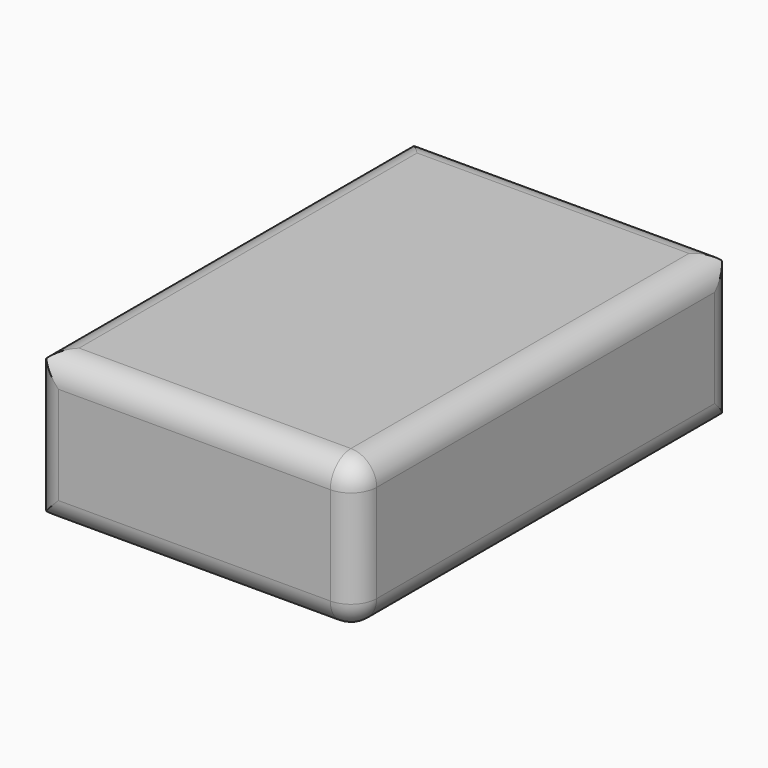
from build123d import *

# Parameters (mm, degrees)
F0_W        = 63.7673679739
F0_H        = 29.4773685746
F1_DEPTH    = 93.472
F2_R        = 5.08
F3_T1_DEPTH = 113.792
F3_T3_DEPTH = 54.8773685746
F4_T1_DEPTH = 79.007367974


# Not quite as in the source:
# - a fillet or chamfer that OpenCascade refuses, or shapes differently, is made with other operations: its cross-section is extruded or revolved along the edge and cut away or added
# - the program builds the solid bodies; features that only make, move or delete a surface that nothing else refers to are left out


with BuildPart() as f1:
    # F0 (on Front) → F1 (new body)
    with BuildSketch(Plane.XZ):
        with Locations((-3.0078953132, 7.5197371189)):
            Rectangle(F0_W, F0_H)
    extrude(amount=F1_DEPTH)

    # F2
    f2_edges = [f1.edges().sort_by_distance(p)[0] for p in [
        (-3.007895, -93.472, 22.258421),
        (-34.891579, -93.472, 7.519737),
        (-3.007895, -93.472, -7.218947),
        (28.875789, -93.472, 7.519737),
        (28.875789, -46.736, -7.218947),
        (28.875789, -46.736, 22.258421),
        (28.875789, 0, 7.519737),
    ]]
    fillet(f2_edges, radius=F2_R)

    # F3: fillet of radius 5.08 on 4 edges, made by hand

    # F3_s2 → F3_t1 (cut)
    with BuildSketch(Plane.XZ.offset(-12.7)):
        with BuildLine():
            ThreePointArc((-29.8115793002, 22.2584214061), (-33.4036817486, 20.7705238546), (-34.8915793002, 17.1784214061))
            Line((-34.8915793002, 17.1784214061), (-34.8915793002, 22.2584214061))
            Line((-34.8915793002, 22.2584214061), (-29.8115793002, 22.2584214061))
        make_face()
        with BuildLine():
            ThreePointArc((-34.8915793002, -2.1389471684), (-33.4036817486, -5.7310496169), (-29.8115793002, -7.2189471684))
            Line((-29.8115793002, -7.2189471684), (-34.8915793002, -7.2189471684))
            Line((-34.8915793002, -7.2189471684), (-34.8915793002, -2.1389471684))
        make_face()
    extrude(amount=F3_T1_DEPTH, mode=Mode.SUBTRACT)

    # F3_s4 → F3_t3 (cut)
    with BuildSketch(Plane.XY.offset(-19.9189471684)):
        with BuildLine():
            ThreePointArc((-34.8915793002, -5.08), (-33.4036817486, -1.4878975516), (-29.8115793002, 0))
            Line((-29.8115793002, 0), (-34.8915793002, 0))
            Line((-34.8915793002, 0), (-34.8915793002, -5.08))
        make_face()
    extrude(amount=F3_T3_DEPTH, mode=Mode.SUBTRACT)

    # F4: fillet of radius 5.08 on 4 edges, made by hand

    # F4_s2 → F4_t1 (cut)
    with BuildSketch(Plane.YZ.offset(-42.5115793002)):
        with BuildLine():
            ThreePointArc((0, -2.1389471684), (-1.4878975516, -5.7310496169), (-5.08, -7.2189471684))
            Line((-5.08, -7.2189471684), (0, -7.2189471684))
            Line((0, -7.2189471684), (0, -2.1389471684))
        make_face()
        with BuildLine():
            ThreePointArc((-5.08, 22.2584214061), (-1.4878975516, 20.7705238546), (0, 17.1784214061))
            Line((0, 17.1784214061), (0, 22.2584214061))
            Line((0, 22.2584214061), (-5.08, 22.2584214061))
        make_face()
    extrude(amount=F4_T1_DEPTH, mode=Mode.SUBTRACT)


solid = f1.part
